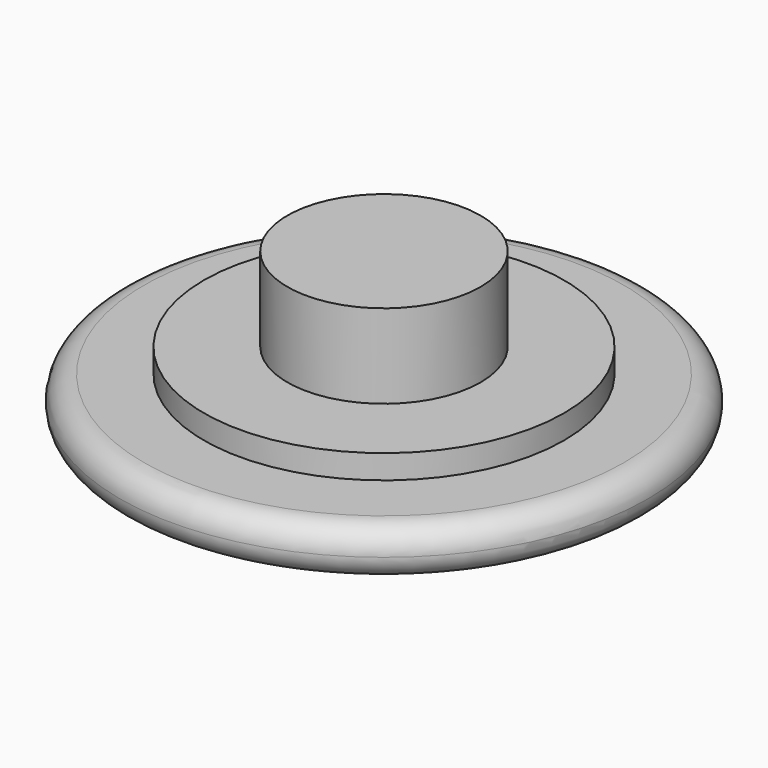
from build123d import *

# Parameters (mm, degrees)
F0_R     = 4.025
F1_DEPTH = 6.5
F0_R_2   = 7.5
F2_DEPTH = 3
F0_R_3   = 11
F3_DEPTH = 2
F4_R     = 0.99999


# Not quite as in the source:
# - a fillet or chamfer is up to 0.001 mm smaller than in the source, because OpenCascade refuses the exact size


with BuildPart() as f1:
    # F0 (on Top) → F1 (new body)
    with BuildSketch(Plane.XY):
        Circle(F0_R)
    extrude(amount=F1_DEPTH)

    # F0 (on Top) → F2 (join)
    with BuildSketch(Plane.XY):
        Circle(F0_R_2)
        Circle(F0_R, mode=Mode.SUBTRACT)
    extrude(amount=F2_DEPTH)

    # F0 (on Top) → F3 (join)
    with BuildSketch(Plane.XY):
        Circle(F0_R_3)
        Circle(F0_R_2, mode=Mode.SUBTRACT)
    extrude(amount=F3_DEPTH)

    # F4 (radius 1 in the source; OpenCascade refuses exactly that, so slightly less here)
    f4_edges = [f1.edges().sort_by_distance(p)[0] for p in [
        (-11, 0, 2),
        (-11, 0, 0),
    ]]
    fillet(f4_edges, radius=F4_R)


solid = f1.part
